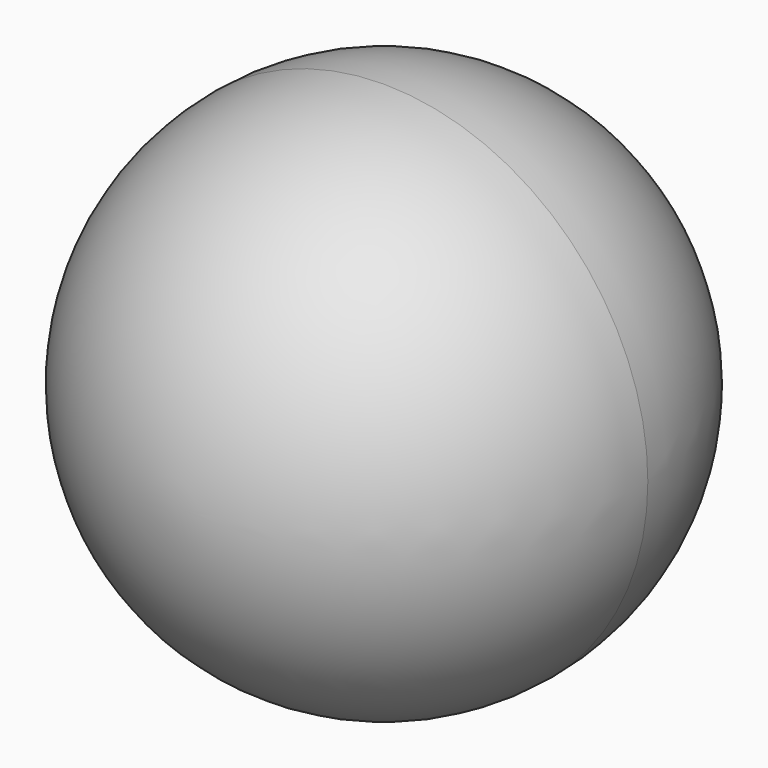
from build123d import *


with BuildPart() as f2:
    # F0 (on Top) → F2 (revolve)
    with BuildSketch(Plane.XY):
        with BuildLine():
            ThreePointArc((0, -1.27), (0.8980256121, -0.8980256121), (1.27, 0))
            ThreePointArc((1.27, 0), (0.8980256121, 0.8980256121), (0, 1.27))
            Line((0, 1.27), (0, 0))
            Line((0, 0), (0, -1.27))
        make_face()
    revolve(axis=Axis((0, 0.030922005, 0), (0, 1, 0)))


solid = f2.part
